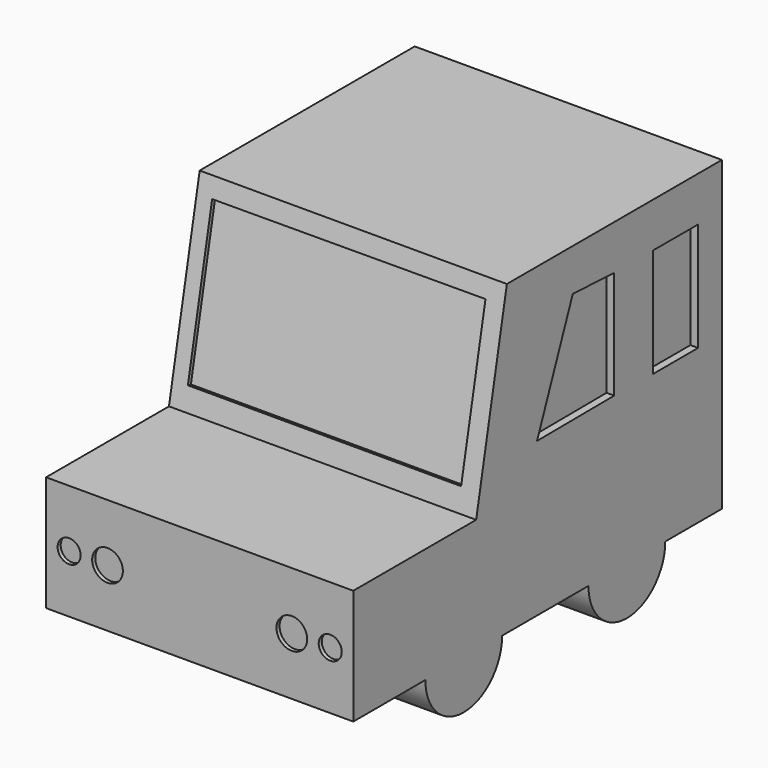
from build123d import *

# Parameters (mm, degrees)
F1_DEPTH = 40
F2_W     = 14.6631337702
F2_H     = 28.3150114119
F3_DEPTH = 2
F5_DEPTH = 1
F6_R     = 3
F6_R_2   = 4
F7_DEPTH = 1


# Not quite as in the source:
# - a pattern or mirror of a feature is missing from the dataset's text; its kind, count and spacing are read off the source's solid


with BuildPart() as f1:
    # F0 (on Right) → F1 (new body, symmetric)
    with BuildSketch(Plane.YZ):
        with BuildLine():
            Line((74.1590947979, 0), (74.1590947979, 80))
            Line((74.1590947979, 80), (4.1590947979, 80))
            Line((4.1590947979, 80), (-5.8409052021, 30))
            Line((-5.8409052021, 30), (-45.8409052021, 30))
            Line((-45.8409052021, 30), (-45.8409052021, 0))
            Line((-45.8409052021, 0), (-22.3770336471, 0))
            ThreePointArc((-22.3770336471, 0), (-9.8770336471, 12.5), (2.6229663529, 0))
            Line((2.6229663529, 0), (30.7202589484, 0))
            ThreePointArc((30.7202589484, 0), (43.2202589484, 12.5), (55.7202589484, 0))
            Line((55.7202589484, 0), (74.1590947979, 0))
        make_face()
        with BuildLine():
            ThreePointArc((30.7202589484, 0), (43.2202589484, -12.5), (55.7202589484, 0))
            Line((55.7202589484, 0), (30.7202589484, 0))
        make_face()
        with BuildLine():
            Line((30.7202589484, 0), (55.7202589484, 0))
            ThreePointArc((55.7202589484, 0), (43.2202589484, 12.5), (30.7202589484, 0))
        make_face()
        with BuildLine():
            ThreePointArc((-22.3770336471, 0), (-9.8770336471, -12.5), (2.6229663529, 0))
            Line((2.6229663529, 0), (-22.3770336471, 0))
        make_face()
        with BuildLine():
            Line((-22.3770336471, 0), (2.6229663529, 0))
            ThreePointArc((2.6229663529, 0), (-9.8770336471, 12.5), (-22.3770336471, 0))
        make_face()
    extrude(amount=F1_DEPTH, both=True)

    # F2 (on face) → F3 (cut)
    with BuildSketch(Plane(origin=(-40, 0, 0), x_dir=(0, -1, 0), z_dir=(-1, 0, 0))):
        Polygon((-13.9850862324, 40.0354526937), (-25.6144665182, 69.0246298909), (-39.0978083014, 68.3504641056), (-39.0978083014, 40.2039922774), align=None)
        with Locations((-59.0700041503, 54.1929583997)):
            Rectangle(F2_W, F2_H)
    f3 = extrude(amount=-F3_DEPTH, mode=Mode.SUBTRACT)

    # F3_copies: F3 across plane
    add(f3.mirror(Plane(origin=(0, 0, 0), x_dir=(0, 0, 1), z_dir=(1, 0, 0))), mode=Mode.SUBTRACT)

    # F4 (on face) → F5 (cut, symmetric)
    with BuildSketch(Plane(origin=(0, -11.3854857713, 2.2770971543), x_dir=(1, 0, 0), z_dir=(0, -0.9805806757, 0.1961161351))):
        Polygon((35.1756438613, 74.5268389583), (-35.977371037, 74.3224471807), (-35.977371037, 34.0555720031), (35.1756438613, 34.0555720031), align=None)
    extrude(amount=F5_DEPTH, both=True, mode=Mode.SUBTRACT)

    # F6 (on face) → F7 (cut, symmetric)
    with BuildSketch(Plane.XZ.offset(45.8409052021)):
        with Locations((-34, 15)):
            Circle(F6_R)
        with Locations((-24, 15)):
            Circle(F6_R_2)
        with Locations((24, 15)):
            Circle(F6_R_2)
        with Locations((34, 15)):
            Circle(F6_R)
    extrude(amount=F7_DEPTH, both=True, mode=Mode.SUBTRACT)


solid = f1.part
